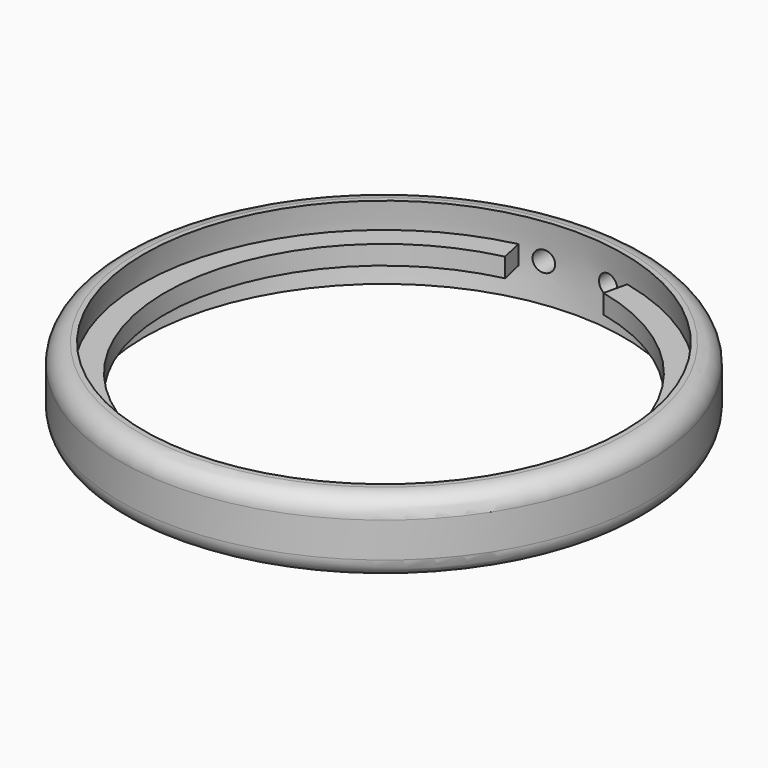
from build123d import *

# Parameters (mm, degrees)
F5_R           = 2
F1_R           = 1.0708620531
F6_DEPTH       = 43.9
F7_ANGLE_START = 100
F7_ANGLE       = 157
F8_ANGLE_BACK  = 77
F8_ANGLE       = 177
F9_DEPTH       = 25


with BuildPart() as f2:
    # F1 (on Front) → F2 (revolve)
    with BuildSketch(Plane.XZ):
        with BuildLine():
            ThreePointArc((-25.1082326719, -3.8388347315), (-25.4, 0), (-25.1082326719, 3.8388347315))
            Line((-25.1082326719, 3.8388347315), (-27.6482326719, 3.8388347315))
            Line((-27.6482326719, 3.8388347315), (-27.6482326719, -3.8388347315))
            Line((-27.6482326719, -3.8388347315), (-25.1082326719, -3.8388347315))
        make_face()
    revolve(axis=Axis((0, 0, 0.0089984387), (0, 0, -1)))

    # F5
    f5_edges = [f2.edges().sort_by_distance(p)[0] for p in [
        (27.648233, 0, 3.838835),
        (27.648233, 0, -3.838835),
    ]]
    fillet(f5_edges, radius=F5_R)

    # F1 (on Front) → F6 (cut)
    with BuildSketch(Plane.XZ):
        with Locations((3.3717958722, 0)):
            Circle(F1_R)
        with Locations((-3.3717958722, 0)):
            Circle(F1_R)
    extrude(amount=-F6_DEPTH, mode=Mode.SUBTRACT)

    # F1 (on Front) → F7 (revolve)
    with BuildSketch(Plane.XZ, mode=Mode.PRIVATE) as f7_sk:
        with BuildLine():
            ThreePointArc((25.3803073267, -1), (25.3950763545, -0.5000969409), (25.4, 0))
            ThreePointArc((25.4, 0), (25.3950763545, 0.5000969409), (25.3803073267, 1))
            Line((25.3803073267, 1), (22.9, 1))
            Line((22.9, 1), (22.9, -1))
            Line((22.9, -1), (25.3803073267, -1))
        make_face()
    revolve(f7_sk.sketch.rotate(Axis((0, 0, 0.0089984387), (0, 0, -1)), F7_ANGLE_START), axis=Axis((0, 0, 0.0089984387), (0, 0, -1)), revolution_arc=F7_ANGLE)

    # F1 (on Front) → F8 (revolve)
    with BuildSketch(Plane.XZ, mode=Mode.PRIVATE) as f8_sk:
        with BuildLine():
            ThreePointArc((25.3803073267, -1), (25.3950763545, -0.5000969409), (25.4, 0))
            ThreePointArc((25.4, 0), (25.3950763545, 0.5000969409), (25.3803073267, 1))
            Line((25.3803073267, 1), (22.9, 1))
            Line((22.9, 1), (22.9, -1))
            Line((22.9, -1), (25.3803073267, -1))
        make_face()
    revolve(f8_sk.sketch.rotate(Axis((0, 0, 0.0089984387), (0, 0, -1)), -F8_ANGLE_BACK), axis=Axis((0, 0, 0.0089984387), (0, 0, -1)), revolution_arc=F8_ANGLE)

    # F1 (on Front) → F9 (cut)
    with BuildSketch(Plane.XZ):
        with BuildLine():
            Line((0, -0.700821599), (0, 0.700821599))
            ThreePointArc((0, 0.700821599), (-0.700821599, 0), (0, -0.700821599))
        make_face()
        with BuildLine():
            ThreePointArc((0.700821599, 0), (0.4955557051, 0.4955557051), (0, 0.700821599))
            Line((0, 0.700821599), (0, -0.700821599))
            ThreePointArc((0, -0.700821599), (0.4955557051, -0.4955557051), (0.700821599, 0))
        make_face()
    extrude(amount=F9_DEPTH, mode=Mode.SUBTRACT)


solid = f2.part
